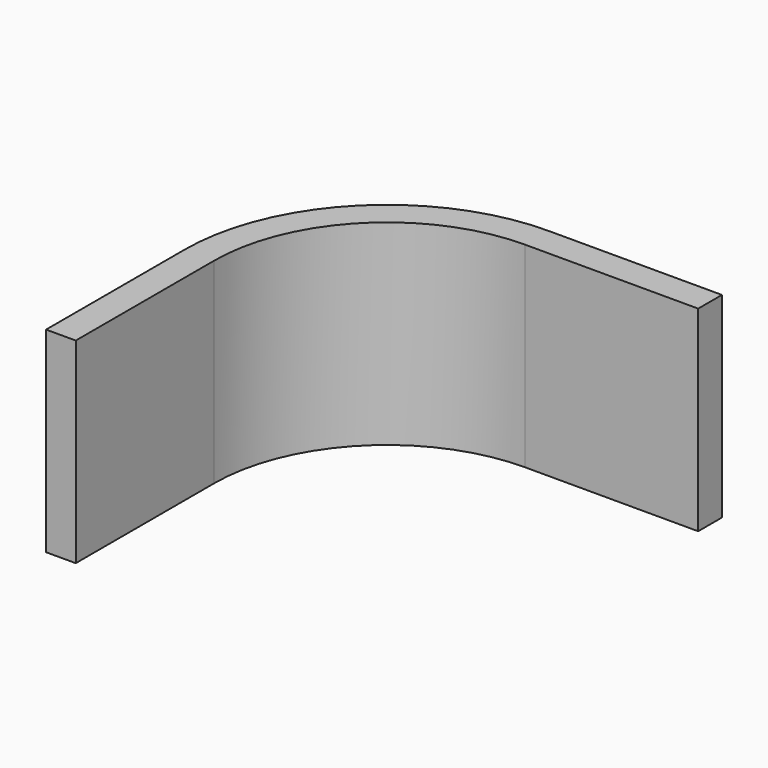
from build123d import *

# Parameters (mm, degrees)
F0_R     = 35.128120954
F0_R_2   = 29.9814765583
F1_DEPTH = 34
F3_DEPTH = 56.7
F4_DEPTH = 15
F5_DEPTH = 15
F6_DEPTH = 15
F7_DEPTH = 15


# Not quite as in the source:
# - a feature names something its author has since deleted; it is built from what else it names


with BuildPart() as f1:
    # F0 (on Top) → F1 (new body)
    with BuildSketch(Plane.XY):
        Circle(F0_R)
        Circle(F0_R_2, mode=Mode.SUBTRACT)
    extrude(amount=F1_DEPTH)

    # F2 (on Top) → F3 (cut)
    with BuildSketch(Plane.XY):
        Polygon((0, 50.666205585), (0, 0), (-44.6641780436, 0), (-44.6641780436, -44.4084256887), (0, -44.4084256887), (0, -49.6323108673), (44.1417917609, -49.6323108673), (44.1417917609, 0), (47.7985069156, 0), (47.7985069156, 50.666205585), align=None)
    extrude(amount=F3_DEPTH, mode=Mode.SUBTRACT)

    # F4 (add): a face of the model
    f4_faces = [f1.faces().sort_by_distance(p)[0] for p in [
        (0, 32.5547987561, 17),
    ]]
    extrude(f4_faces, amount=F4_DEPTH)

    # F5 (add): a face of the model
    f5_faces = [f1.faces().sort_by_distance(p)[0] for p in [
        (-32.5547987561, 0, 17),
    ]]
    extrude(f5_faces, amount=F5_DEPTH)

    # F6 (add): a face of the model
    f6_faces = [f1.faces().sort_by_distance(p)[0] for p in [
        (-32.5547987561, -15, 17),
    ]]
    extrude(f6_faces, amount=F6_DEPTH)

    # F7 (add): a face of the model
    f7_faces = [f1.faces().sort_by_distance(p)[0] for p in [
        (15, 32.5547987561, 17),
    ]]
    extrude(f7_faces, amount=F7_DEPTH)


solid = f1.part
